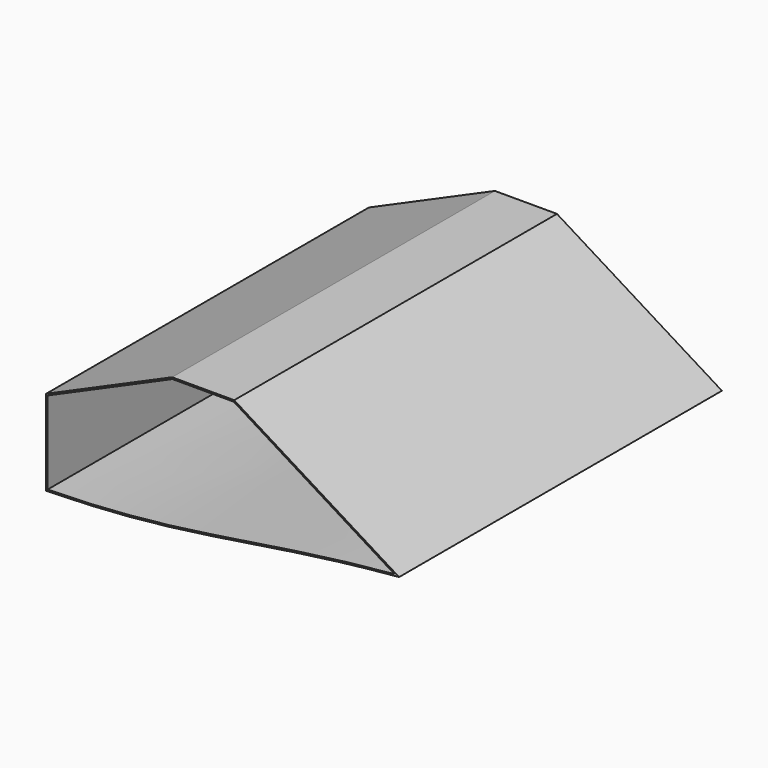
from build123d import *

# Parameters (mm, degrees)
F1_DEPTH = 528.32


# Not quite as in the source:
# - ends of sketch curves that miss each other by under 0.0002 mm in the source are joined


with BuildPart() as f1:
    # F0 (on Front) → F1 (new body)
    with BuildSketch(Plane.XZ):
        with BuildLine():
            Line((-209.5452234585, 27.1872572403), (-209.5452234585, -84.5727427597))
            add(Edge.make_bspline(
                [(-209.5452234585, -84.5727427597), (-19.6203030646, -81.5465301275), (60.0399486721, -50.63669011), (252.7347765415, -33.7727427597)],
                knots=[0, 0, 0, 0, 465.0628327441, 465.0628327441, 465.0628327441, 465.0628327441], degree=3))
            Line((252.7347765415, -33.7727427597), (36.7612242285, 99.9113052838))
            Line((36.7612242285, 99.9113052838), (-44.5187757715, 99.9113052838))
            Line((-44.5187757715, 99.9113052838), (-209.5452234585, 27.1872572403))
        make_face()
        with BuildLine():
            Line((-44.0976344097, 97.9113052838), (36.192323926, 97.9113052838))
            Line((36.192323926, 97.9113052838), (246.5747366709, -32.311920068))
            add(Edge.make_bspline(
                [(-207.545223454, -82.5394870183), (-160.9885784093, -81.7456194303), (-80.6027101112, -76.7587307387), (20.1465558538, -62.8204704396), (120.6324842882, -46.4287449505), (200.9255170344, -36.424903597), (246.5747366709, -32.311920068)],
                knots=[0.003577419, 0.003577419, 0.003577419, 0.003577419, 0.25, 0.5, 0.75, 0.9895914005, 0.9895914005, 0.9895914005, 0.9895914005], degree=3))
            Line((-207.545223454, -82.5394870183), (-207.5452234585, 25.8830305123))
            Line((-207.5452234585, 25.8830305123), (-44.0976344097, 97.9113052838))
        make_face(mode=Mode.SUBTRACT)
    extrude(amount=F1_DEPTH)


solid = f1.part
